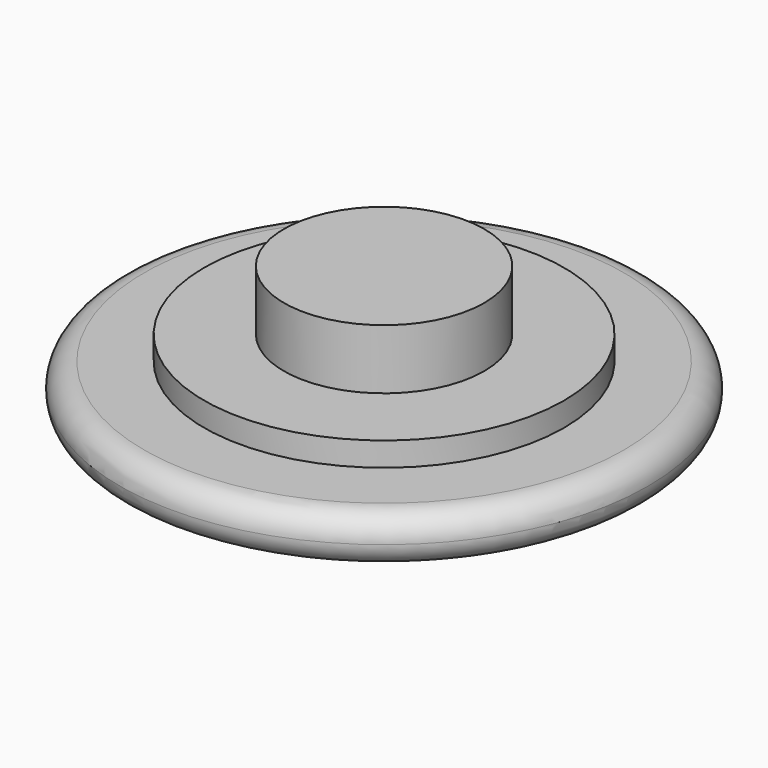
from build123d import *

# Parameters (mm, degrees)
F0_R         = 11
F0_R_2       = 7.5
F1_DEPTH     = 2
F0_R_3       = 4.175
F2_DEPTH     = 3
F3_DEPTH     = 5.5
F4_R         = 0.99999
F5_TEXT_SIZE = 6.49886791
F6_DEPTH     = 1


# Not quite as in the source:
# - a fillet or chamfer is up to 0.001 mm smaller than in the source, because OpenCascade refuses the exact size
# - Text() gives the source's letters only with a copy of the font that has no kerning and outlines rounded to 1/6400 em; it was checked with that copy


with BuildPart() as f1:
    # F0 (on Top) → F1 (new body)
    with BuildSketch(Plane.XY):
        Circle(F0_R)
        Circle(F0_R_2, mode=Mode.SUBTRACT)
    extrude(amount=F1_DEPTH)

    # F0 (on Top) → F2 (join)
    with BuildSketch(Plane.XY):
        Circle(F0_R_2)
        Circle(F0_R_3, mode=Mode.SUBTRACT)
    extrude(amount=F2_DEPTH)

    # F0 (on Top) → F3 (join)
    with BuildSketch(Plane.XY):
        Circle(F0_R_3)
    extrude(amount=F3_DEPTH)

    # F4 (radius 1 in the source; OpenCascade refuses exactly that, so slightly less here)
    f4_edges = [f1.edges().sort_by_distance(p)[0] for p in [
        (-11, 0, 2),
        (-11, 0, 0),
    ]]
    fillet(f4_edges, radius=F4_R)

    # F5 (on face) → F6 (cut)
    with BuildSketch(Plane(origin=(0, 0, 0), x_dir=(1, 0, 0), z_dir=(0, 0, -1))):
        with Locations((-9.7551666572, -2.1992552126)):
            Text('Linsey', F5_TEXT_SIZE, font='Open Sans', text_align=(TextAlign.LEFT, TextAlign.BOTTOM))
    extrude(amount=-F6_DEPTH, mode=Mode.SUBTRACT)


solid = f1.part
